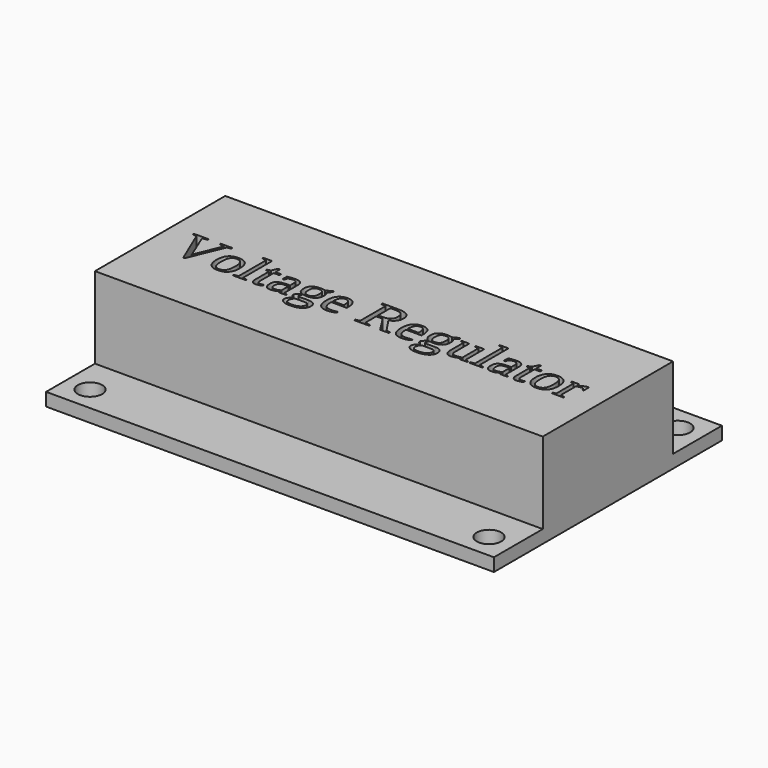
from build123d import *

# Parameters (mm, degrees)
F0_W         = 55
F0_H         = 35
F0_R         = 1.5
F1_DEPTH     = 1.6
F2_W         = 55
F2_H         = 20
F3_DEPTH     = 10
F4_TEXT_SIZE = 6.7450782008
F5_DEPTH     = 3


# Not quite as in the source:
# - Text() gives the source's letters only with a copy of the font that has no kerning and outlines rounded to 1/6400 em; it was checked with that copy


with BuildPart() as f1:
    # F0 (on Top) → F1 (new body)
    with BuildSketch(Plane.XY):
        Rectangle(F0_W, F0_H)
        with Locations((-24.5, -14.5)):
            Circle(F0_R, mode=Mode.SUBTRACT)
        with Locations((24.5, -14.5)):
            Circle(F0_R, mode=Mode.SUBTRACT)
        with Locations((-24.5, 14.5)):
            Circle(F0_R, mode=Mode.SUBTRACT)
        with Locations((24.5, 14.5)):
            Circle(F0_R, mode=Mode.SUBTRACT)
    extrude(amount=F1_DEPTH)

    # F2 (on face) → F3 (join)
    with BuildSketch(Plane.XY.offset(1.6)):
        Rectangle(F2_W, F2_H)
    extrude(amount=F3_DEPTH)

    # F4 (on face) → F5 (cut)
    with BuildSketch(Plane.XY.offset(11.6)):
        with Locations((-25, -2.4282281523)):
            Text('Voltage Regulator', F4_TEXT_SIZE, font='Tinos', text_align=(TextAlign.LEFT, TextAlign.BOTTOM))
    extrude(amount=-F5_DEPTH, mode=Mode.SUBTRACT)


solid = f1.part
